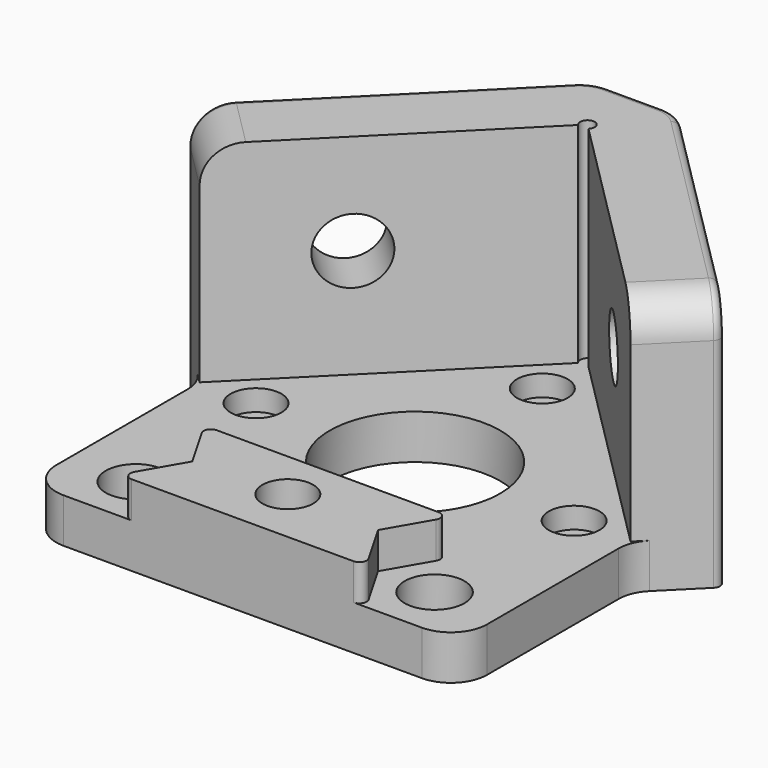
from build123d import *

# Parameters (mm, degrees)
F0_R          = 4.125
F0_R_2        = 1.7
F0_R_3        = 11.75
F1_DEPTH      = 6.13
F3_DEPTH      = 35
F4_R          = 4.5
F5_DEPTH      = 10
F6_R          = 4.25
F7_DEPTH      = 10
F8_R          = 7
F9_DEPTH      = 3
F10_R         = 7
F11_DEPTH     = 3
F13_R         = 5
F12_R         = 3.5
F14_DEPTH     = 2.9
F15_TEXT_SIZE = 7.1642815932
F16_DEPTH     = 0.25
F17_R         = 3.5
F18_DEPTH     = 5
F19_T1_DEPTH  = 32.5
F19_T3_DEPTH  = 9.3301270189
F19_T5_DEPTH  = 36.6690475583
F19_T7_DEPTH  = 7.5391052434
F19_T9_DEPTH  = 36.6690475583
F19_T12_ANGLE = 90
F19_T14_ANGLE = 45
F19_T16_ANGLE = 45
F19_T18_ANGLE = 90
F20_R         = 1
F21_DEPTH     = 28.87


# Not quite as in the source:
# - a fillet or chamfer that OpenCascade refuses, or shapes differently, is made with other operations: its cross-section is extruded or revolved along the edge and cut away or added
# - Text() gives the source's letters only with a copy of the font that has no kerning and outlines rounded to 1/6400 em; it was checked with that copy


with BuildPart() as f1:
    # F0 (on Top) → F1 (new body)
    with BuildSketch(Plane.XY):
        Polygon((-29.6984848098, 0), (0, 0), (29.6984848098, 0), (29.6984848098, 29.7), (0, 59.3984848098), (-29.6984848098, 29.7), align=None)
        with Locations((-20.59, 7.3196897832)):
            Circle(F0_R, mode=Mode.SUBTRACT)
        with Locations((0, 7.7796897832)):
            Circle(F0_R_2, mode=Mode.SUBTRACT)
        with Locations((20.59, 7.3196897832)):
            Circle(F0_R, mode=Mode.SUBTRACT)
        with Locations((-21.9203102168, 29.7)):
            Circle(F0_R_2, mode=Mode.SUBTRACT)
        with Locations((0, 29.7)):
            Circle(F0_R_3, mode=Mode.SUBTRACT)
        with Locations((21.9203102168, 29.7)):
            Circle(F0_R_2, mode=Mode.SUBTRACT)
        with Locations((0, 51.6203102168)):
            Circle(F0_R_2, mode=Mode.SUBTRACT)
    extrude(amount=F1_DEPTH)

    # F2 (on face) → F3 (join)
    with BuildSketch(Plane(origin=(0, 0, 0), x_dir=(1, 0, 0), z_dir=(0, 0, -1))):
        Polygon((0, -59.3984848098), (-29.6984848098, -29.7), (-36.7695526217, -36.7710678119), (-5.8406204336, -67.7), (0, -67.7), (5.8406204336, -67.7), (36.7695526217, -36.7710678119), (29.6984848098, -29.7), align=None)
    extrude(amount=-F3_DEPTH)

    # F4 (on face) → F5 (cut, through all)
    with BuildSketch(Plane(origin=(-29.6992424049, 29.6992424049, 0), x_dir=(0.7071067812, 0.7071067812, 0), z_dir=(0.7071067812, -0.7071067812, 0))):
        with Locations((16.6010714012, 21.13)):
            Circle(F4_R)
    extrude(amount=-F5_DEPTH, mode=Mode.SUBTRACT)

    # F6 (on face) → F7 (cut, through all)
    with BuildSketch(Plane(origin=(29.6992424049, 29.6992424049, 0), x_dir=(0.7071067812, -0.7071067812, 0), z_dir=(-0.7071067812, -0.7071067812, 0))):
        with Locations((-16.6010714012, 21.13)):
            Circle(F6_R)
    extrude(amount=-F7_DEPTH, mode=Mode.SUBTRACT)

    # F8 (on face) → F9 (cut)
    with BuildSketch(Plane(origin=(-36.7703102168, 36.7703102168, 0), x_dir=(-0.7071067812, -0.7071067812, 0), z_dir=(-0.7071067812, 0.7071067812, 0))):
        with Locations((-16.6010714005, 21.13)):
            Circle(F8_R)
    extrude(amount=-F9_DEPTH, mode=Mode.SUBTRACT)

    # F10 (on face) → F11 (cut)
    with BuildSketch(Plane(origin=(36.7703102168, 36.7703102168, 0), x_dir=(-0.7071067812, 0.7071067812, 0), z_dir=(0.7071067812, 0.7071067812, 0))):
        with Locations((16.6010714006, 21.13)):
            Circle(F10_R)
    extrude(amount=-F11_DEPTH, mode=Mode.SUBTRACT)

    # F13
    f13_edges = [f1.edges().sort_by_distance(p)[0] for p in [
        (33.234019, 33.235534, 35),
        (-33.234019, 33.235534, 35),
        (29.698485, 29.7, 3.065),
        (29.698485, 0, 3.065),
        (-29.698485, 0, 3.065),
        (-29.698485, 29.7, 3.065),
        (-5.84062, 67.7, 17.5),
        (5.84062, 67.7, 17.5),
    ]]
    fillet(f13_edges, radius=F13_R)

    # F12 (on face) → F14 (cut)
    with BuildSketch(Plane.XY.offset(6.13)):
        with Locations((0, 51.6203102168)):
            Circle(F12_R)
        with Locations((-21.9203102168, 29.7)):
            Circle(F12_R)
        with Locations((21.9203102168, 29.7)):
            Circle(F12_R)
        with Locations((0, 7.7796897832)):
            Circle(F12_R)
    extrude(amount=-F14_DEPTH, mode=Mode.SUBTRACT)

    # F15 (on face) → F16 (cut)
    with BuildSketch(Plane(origin=(-36.7703102168, 36.7703102168, 0), x_dir=(-0.7071067812, -0.7071067812, 0), z_dir=(-0.7071067812, 0.7071067812, 0))):
        with Locations((-41.6701189596, 3.2)):
            Text('SIENCI LABS', F15_TEXT_SIZE, font='Open Sans', text_align=(TextAlign.LEFT, TextAlign.BOTTOM))
    extrude(amount=-F16_DEPTH, mode=Mode.SUBTRACT)

    # F17 (on face) → F18 (join)
    with BuildSketch(Plane.XY.offset(6.13)):
        Polygon((16.692885683, 14.0696897832), (-16.692885683, 14.0696897832), (-12.7957713659, 7.3196897832), (-16.692885683, 0.5696897832), (16.692885683, 0.5696897832), (12.7957713659, 7.3196897832), align=None)
        with Locations((0, 7.7796897832)):
            Circle(F17_R, mode=Mode.SUBTRACT)
        Polygon((16.692885683, 0.5696897832), (-16.692885683, 0.5696897832), (-17.0217962327, 0), (0, 0), (17.0217962327, 0), align=None)
        Polygon((-17.0217962327, 14.6393795664), (-16.692885683, 14.0696897832), (16.692885683, 14.0696897832), (17.0217962327, 14.6393795664), (0, 14.6393795664), align=None)
    extrude(amount=F18_DEPTH)

    # F19: fillet of radius 1 on 13 edges, made by hand

    # F19_s2 → F19_t1 (cut)
    with BuildSketch(Plane.XY.offset(-2.5)):
        with BuildLine():
            ThreePointArc((36.0624458405, 37.4781745931), (36.3553390593, 36.7710678119), (36.0624458405, 36.0639610307))
            Line((36.0624458405, 36.0639610307), (36.7695526217, 36.7710678119))
            Line((36.7695526217, 36.7710678119), (36.0624458405, 37.4781745931))
        make_face()
        with BuildLine():
            ThreePointArc((-36.0624458405, 36.0639610307), (-36.3553390593, 36.7710678119), (-36.0624458405, 37.4781745931))
            Line((-36.0624458405, 37.4781745931), (-36.7695526217, 36.7710678119))
            Line((-36.7695526217, 36.7710678119), (-36.0624458405, 36.0639610307))
        make_face()
    extrude(amount=F19_T1_DEPTH, mode=Mode.SUBTRACT)

    # F19_s4 → F19_t3 (cut)
    with BuildSketch(Plane.XY.offset(6.13)):
        with BuildLine():
            ThreePointArc((-15.2897454251, 0), (-16.1557708289, 0.5), (-16.1557708289, 1.5))
            Line((-16.1557708289, 1.5), (-17.0217962327, 0))
            Line((-17.0217962327, 0), (-15.2897454251, 0))
        make_face()
        with BuildLine():
            ThreePointArc((-15.2897454251, 14.6393795664), (-16.1557708289, 14.1393795664), (-16.1557708289, 13.1393795664))
            Line((-16.1557708289, 13.1393795664), (-17.0217962327, 14.6393795664))
            Line((-17.0217962327, 14.6393795664), (-15.2897454251, 14.6393795664))
        make_face()
        with BuildLine():
            ThreePointArc((16.1557708289, 13.1393795664), (16.1557708289, 14.1393795664), (15.2897454251, 14.6393795664))
            Line((15.2897454251, 14.6393795664), (17.0217962327, 14.6393795664))
            Line((17.0217962327, 14.6393795664), (16.1557708289, 13.1393795664))
        make_face()
        with BuildLine():
            ThreePointArc((15.2897454251, 0), (16.1557708289, 0.5), (16.1557708289, 1.5))
            Line((16.1557708289, 1.5), (17.0217962327, 0))
            Line((17.0217962327, 0), (15.2897454251, 0))
        make_face()
    extrude(amount=F19_T3_DEPTH, mode=Mode.SUBTRACT)

    # F19_s6 → F19_t5 (cut)
    with BuildSketch(Plane(origin=(3.536291501, 3.536291501, 0), x_dir=(0, 0, 1), z_dir=(0.7071067812, 0.7071067812, 0))):
        with BuildLine():
            ThreePointArc((34, -52.0010714012), (34.7071067812, -51.7081781824), (35, -51.0010714012))
            Line((35, -51.0010714012), (35, -52.0010714012))
            Line((35, -52.0010714012), (34, -52.0010714012))
        make_face()
    extrude(amount=F19_T5_DEPTH, mode=Mode.SUBTRACT)

    # F19_s8 → F19_t7 (cut)
    with BuildSketch(Plane.YZ.offset(-3.7695526217)):
        with BuildLine():
            ThreePointArc((67.7, 34), (67.4071067812, 34.7071067812), (66.7, 35))
            Line((66.7, 35), (67.7, 35))
            Line((67.7, 35), (67.7, 34))
        make_face()
    extrude(amount=F19_T7_DEPTH, mode=Mode.SUBTRACT)

    # F19_s10 → F19_t9 (cut)
    with BuildSketch(Plane(origin=(-29.4652236891, 29.4652236891, 0), x_dir=(0, 0, 1), z_dir=(0.7071067812, -0.7071067812, 0))):
        with BuildLine():
            ThreePointArc((34, -52.0010714012), (34.7071067812, -51.7081781824), (35, -51.0010714012))
            Line((35, -51.0010714012), (35, -52.0010714012))
            Line((35, -52.0010714012), (34, -52.0010714012))
        make_face()
    extrude(amount=F19_T9_DEPTH, mode=Mode.SUBTRACT)

    # F19_s11 → F19_t12 (revolve, cut)
    with BuildSketch(Plane.XY.offset(30)):
        with BuildLine():
            ThreePointArc((-36.0624458405, 37.4781745931), (-36.3553390593, 36.7710678119), (-36.0624458405, 36.0639610307))
            Line((-36.0624458405, 36.0639610307), (-36.7695526217, 36.7710678119))
            Line((-36.7695526217, 36.7710678119), (-36.0624458405, 37.4781745931))
        make_face()
    revolve(axis=Axis((-33.2340187158, 40.3066017178, 30), (-0.7071067812, 0.7071067812, 0)), revolution_arc=F19_T12_ANGLE, mode=Mode.SUBTRACT)

    # F19_s13 → F19_t14 (revolve, cut)
    with BuildSketch(Plane.YZ.offset(-3.7695526217)):
        with BuildLine():
            ThreePointArc((67.7, 34), (67.4071067812, 34.7071067812), (66.7, 35))
            Line((66.7, 35), (67.7, 35))
            Line((67.7, 35), (67.7, 34))
        make_face()
    revolve(axis=Axis((-3.7695526217, 62.7, 35), (0, 0, 1)), revolution_arc=F19_T14_ANGLE, mode=Mode.SUBTRACT)

    # F19_s15 → F19_t16 (revolve, cut)
    with BuildSketch(Plane(origin=(-29.4652236891, 29.4652236891, 0), x_dir=(0, 0, 1), z_dir=(0.7071067812, -0.7071067812, 0))):
        with BuildLine():
            ThreePointArc((34, -52.0010714012), (34.7071067812, -51.7081781824), (35, -51.0010714012))
            Line((35, -51.0010714012), (35, -52.0010714012))
            Line((35, -52.0010714012), (34, -52.0010714012))
        make_face()
    revolve(axis=Axis((3.7695526217, 62.7, 35), (0, 0, 1)), revolution_arc=F19_T16_ANGLE, mode=Mode.SUBTRACT)

    # F19_s17 → F19_t18 (revolve, cut)
    with BuildSketch(Plane.XY.offset(30)):
        with BuildLine():
            ThreePointArc((36.0624458405, 37.4781745931), (36.3553390593, 36.7710678119), (36.0624458405, 36.0639610307))
            Line((36.0624458405, 36.0639610307), (36.7695526217, 36.7710678119))
            Line((36.7695526217, 36.7710678119), (36.0624458405, 37.4781745931))
        make_face()
    revolve(axis=Axis((33.2340187158, 40.3066017178, 30), (-0.7071067812, -0.7071067812, 0)), revolution_arc=F19_T18_ANGLE, mode=Mode.SUBTRACT)

    # F20 (on face) → F21 (cut, through all)
    with BuildSketch(Plane.XY.offset(35)):
        with Locations((0, 59.3984848098)):
            Circle(F20_R)
    extrude(amount=-F21_DEPTH, mode=Mode.SUBTRACT)


solid = f1.part
